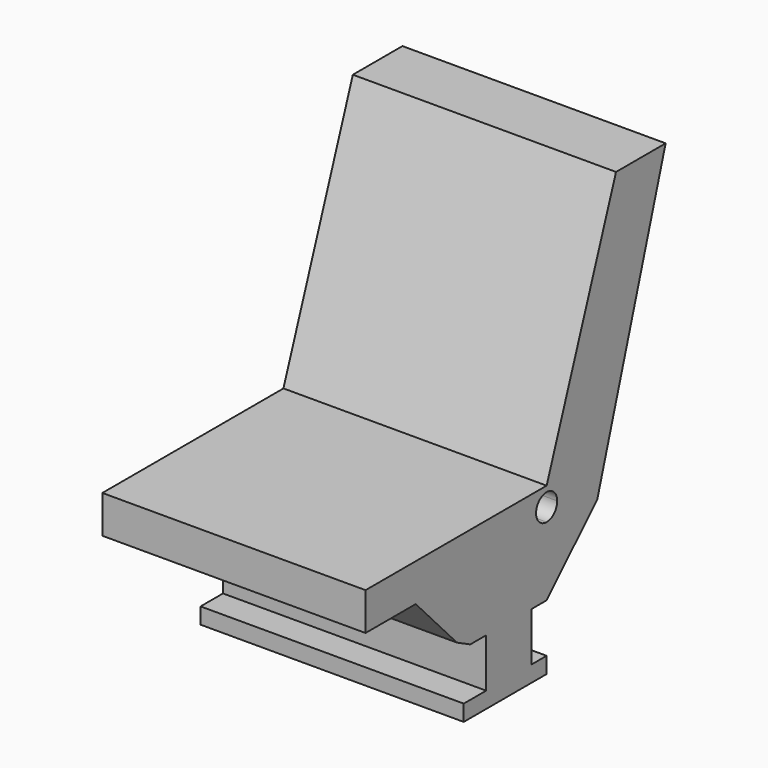
from build123d import *

# Parameters (mm, degrees)
F0_W     = 19.148854
F0_H     = 16.486252
F1_DEPTH = 44.45


with BuildPart() as f1:
    # F0 (on Right) → F1 (new body, symmetric)
    with BuildSketch(Plane.YZ):
        with BuildLine():
            ThreePointArc((0, 4.46964), (3.160513, 3.160513), (4.46964, 0))
            ThreePointArc((4.46964, 0), (3.160513, -3.160513), (0, -4.46964))
            Line((0, -4.46964), (0, -6.37082))
            Line((0, -6.37082), (4.939543, -6.37082))
            Line((4.939543, -6.37082), (21.400414, -6.37082))
            Line((21.400414, -6.37082), (50.244033, 87.741062))
            Line((50.244033, 87.741062), (29.303843, 87.741062))
            Line((29.303843, 87.741062), (0, 6.37082))
            Line((0, 6.37082), (0, 4.46964))
        make_face()
        with BuildLine():
            ThreePointArc((-4.46964, 0), (-3.160513, 3.160513), (0, 4.46964))
            Line((0, 4.46964), (0, 6.37082))
            Line((0, 6.37082), (-4.939543, 6.37082))
            Line((-4.939543, 6.37082), (-76.449834, 6.37082))
            Line((-76.449834, 6.37082), (-76.449834, 0))
            Line((-76.449834, 0), (-4.46964, 0))
        make_face()
        with BuildLine():
            Line((0, -6.37082), (0, -4.46964))
            ThreePointArc((0, -4.46964), (-3.160513, -3.160513), (-4.46964, 0))
            Line((-4.46964, 0), (-76.449834, 0))
            Line((-76.449834, 0), (-76.449834, -6.37082))
            Line((-76.449834, -6.37082), (-55.27623, -6.37082))
            Line((-55.27623, -6.37082), (-4.939543, -6.37082))
            Line((-4.939543, -6.37082), (0, -6.37082))
        make_face()
        Polygon((0, -27.731804), (0, -6.37082), (-4.939543, -6.37082), (-55.27623, -6.37082), (-37.850164, -24.921147), (-32.228854, -27.731804), (-25.522344, -27.731804), (-6.37349, -27.731804), align=None)
        Polygon((4.939543, -6.37082), (0, -6.37082), (0, -27.731804), (21.400414, -6.37082), align=None)
        with Locations((-15.947917, -35.97493)):
            Rectangle(F0_W, F0_H)
        Polygon((0, -44.218056), (-6.37349, -44.218056), (-25.522344, -44.218056), (-34.995988, -44.218056), (-34.995988, -49.660362), (0, -49.660362), align=None)
    extrude(amount=F1_DEPTH, both=True)


solid = f1.part
